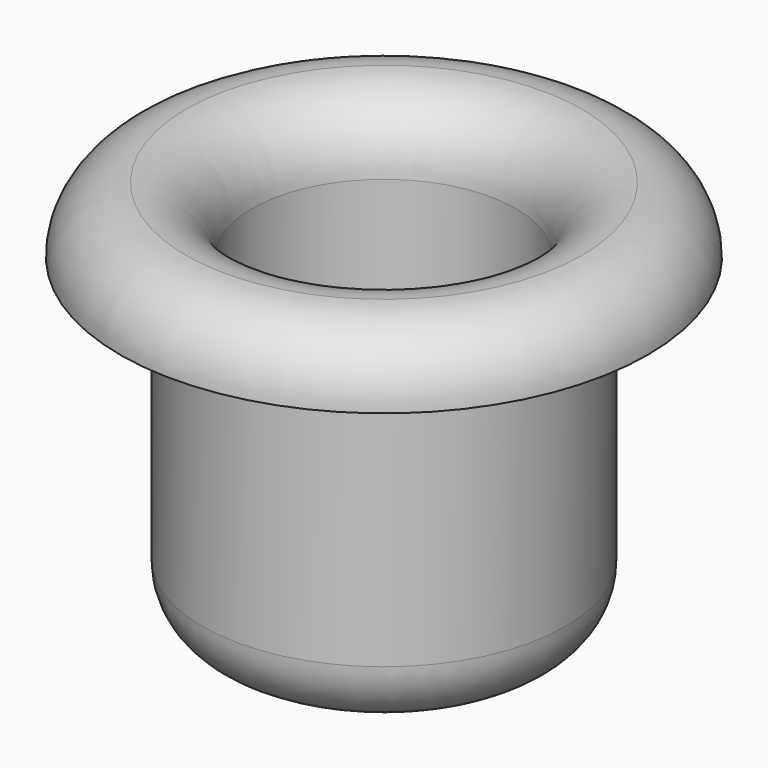
from build123d import *

# Parameters (mm, degrees)
F0_R     = 5.5
F0_R_2   = 4
F1_DEPTH = 10
F0_R_3   = 8
F2_DEPTH = 2


# Not quite as in the source:
# - a fillet or chamfer that OpenCascade refuses, or shapes differently, is made with other operations: its cross-section is extruded or revolved along the edge and cut away or added


with BuildPart() as f1:
    # F0 (on Top) → F1 (new body)
    with BuildSketch(Plane.XY):
        Circle(F0_R)
        Circle(F0_R_2, mode=Mode.SUBTRACT)
    extrude(amount=-F1_DEPTH)

    # F0 (on Top) → F2 (join)
    with BuildSketch(Plane.XY):
        Circle(F0_R_3)
        Circle(F0_R, mode=Mode.SUBTRACT)
        Circle(F0_R)
        Circle(F0_R_2, mode=Mode.SUBTRACT)
    extrude(amount=F2_DEPTH)

    # F3: fillet of radius 2 on 3 edges, made by hand

    # F3_s1 → F3_t2 (revolve, cut)
    with BuildSketch(Plane.XZ):
        with BuildLine():
            ThreePointArc((8, 0), (7.4142135624, 1.4142135624), (6, 2))
            Line((6, 2), (8, 2))
            Line((8, 2), (8, 0))
        make_face()
    revolve(axis=Axis((0, 0, 2), (0, 0, 1)), mode=Mode.SUBTRACT)

    # F3_s3 → F3_t4 (revolve, cut)
    with BuildSketch(Plane.XZ):
        with BuildLine():
            ThreePointArc((6, 2), (4.5857864376, 1.4142135624), (4, 0))
            Line((4, 0), (4, 2))
            Line((4, 2), (6, 2))
        make_face()
    revolve(axis=Axis((0, 0, 2), (0, 0, 1)), mode=Mode.SUBTRACT)

    # F3_s5 → F3_t6 (revolve, cut)
    with BuildSketch(Plane.XZ):
        with BuildLine():
            ThreePointArc((5.5, -8.0635083269), (5.0811388301, -9.2882531983), (4, -10))
            Line((4, -10), (5.5, -10))
            Line((5.5, -10), (5.5, -8.0635083269))
        make_face()
    revolve(axis=Axis((0, 0, -10), (0, 0, 1)), mode=Mode.SUBTRACT)


solid = f1.part
